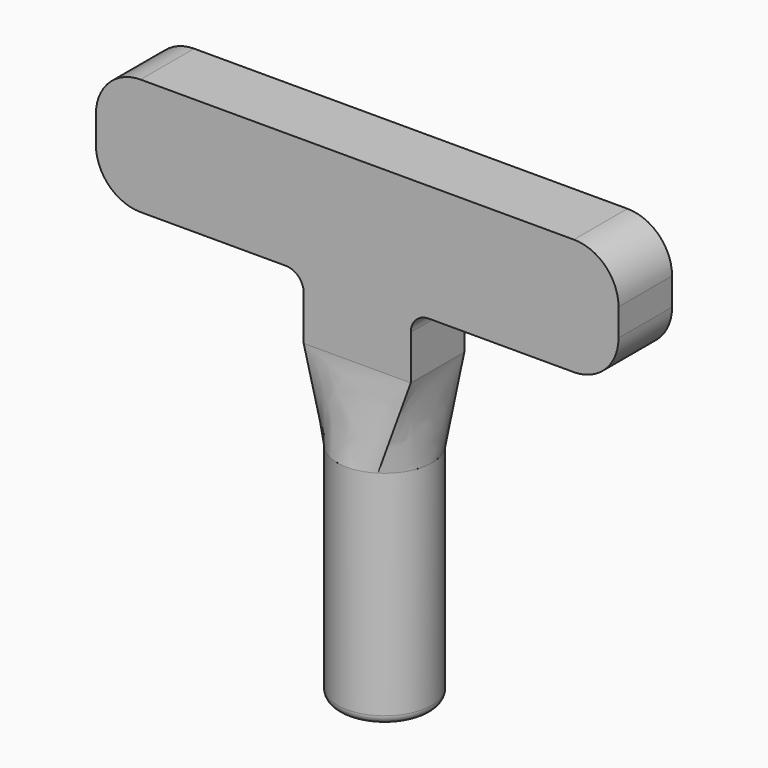
from build123d import *

# Parameters (mm, degrees)
F2_R      = 0.5
F4_DEPTH  = 7.5
F4_FACE_W = 24
F4_FACE_H = 15
F6_R      = 2


# Not quite as in the source:
# - the arcs of a loft's sections are written as splines that run evenly, so that the points pair up as in the source's solid


with BuildPart() as f1:
    # F0 (on Front) → F1 (revolve)
    with BuildSketch(Plane.XZ):
        Polygon((-7.6, -6.539241709), (-7.6, 9.460758291), (0, 9.460758291), (0, 43.2881079614), (-10.6, 43.2881079614), (-10.6, -6.539241709), align=None)
    revolve(axis=Axis((0, 0, 26.3744331262), (0, 0, -1)))

    # F2
    f2_edges = [f1.edges().sort_by_distance(p)[0] for p in [
        (7.6, 0, -6.539242),
    ]]
    fillet(f2_edges, radius=F2_R)

    # F6
    f6_edges = [f1.edges().sort_by_distance(p)[0] for p in [
        (10.6, 0, -6.539242),
        (8.1, 0, -6.539242),
    ]]
    fillet(f6_edges, radius=F6_R)


with BuildPart() as f4:
    # F3 (on Front) → F4 (new body, symmetric)
    with BuildSketch(Plane.XZ):
        with BuildLine():
            Line((-12.1438586622, 62.5112550155), (-0.1438586622, 62.5112550155))
            Line((-0.1438586622, 62.5112550155), (-0.1438586622, 102.6653030368))
            Line((-0.1438586622, 102.6653030368), (-48.6952245638, 102.6653030368))
            ThreePointArc((-48.6952245638, 102.6653030368), (-55.7662923757, 99.7363708486), (-58.6952245638, 92.6653030368))
            Line((-58.6952245638, 92.6653030368), (-58.6952245638, 86.5112550155))
            ThreePointArc((-58.6952245638, 86.5112550155), (-55.7662923757, 79.4401872036), (-48.6952245638, 76.5112550155))
            Line((-48.6952245638, 76.5112550155), (-16.1438586622, 76.5112550155))
            ThreePointArc((-16.1438586622, 76.5112550155), (-13.3154315374, 75.3396821402), (-12.1438586622, 72.5112550155))
            Line((-12.1438586622, 72.5112550155), (-12.1438586622, 62.5112550155))
        make_face()
        with BuildLine():
            Line((-0.1438586622, 102.6653030368), (-0.1438586622, 62.5112550155))
            Line((-0.1438586622, 62.5112550155), (11.8561413378, 62.5112550155))
            Line((11.8561413378, 62.5112550155), (11.8561413378, 72.5112550155))
            ThreePointArc((11.8561413378, 72.5112550155), (13.0277142131, 75.3396821402), (15.8561413378, 76.5112550155))
            Line((15.8561413378, 76.5112550155), (48.4075072394, 76.5112550155))
            ThreePointArc((48.4075072394, 76.5112550155), (55.4785750513, 79.4401872036), (58.4075072394, 86.5112550155))
            Line((58.4075072394, 86.5112550155), (58.4075072394, 92.6653030368))
            ThreePointArc((58.4075072394, 92.6653030368), (55.4785750513, 99.7363708486), (48.4075072394, 102.6653030368))
            Line((48.4075072394, 102.6653030368), (-0.1438586622, 102.6653030368))
        make_face()
    extrude(amount=F4_DEPTH, both=True)

    # F4_face (on face) → F5 section 0
    with BuildSketch(Plane(origin=(-0.1438586622, 0, 62.5112550155), x_dir=(1, 0, 0), z_dir=(0, 0, -1))):
        Rectangle(F4_FACE_W, F4_FACE_H)
    # F1_face (on face) → F5 section 1
    with BuildSketch(Plane.XY.offset(43.2881079614)):
        with BuildLine():
            add(Edge.make_bspline(
                [(8.9581169834, 5.6667574602), (8.2163401664, 6.8393722312), (7.2416993998, 7.8640350998), (4.9735940712, 9.463013276), (3.6810219119, 10.0366994541), (0.9736633644, 10.645996332), (-0.4400577936, 10.6813672994), (-3.1744987633, 10.2082229526), (-4.4941426892, 9.6998938003), (-5.6667574602, 8.9581169834)],
                knots=[0, 0, 0, 0, 0.25, 0.25, 0.5, 0.5, 0.75, 0.75, 1, 1, 1, 1], degree=3))
            add(Edge.make_bspline(
                [(-5.6667574602, 8.9581169834), (-6.8393722312, 8.2163401664), (-7.8640350998, 7.2416993998), (-9.463013276, 4.9735940712), (-10.0366994541, 3.6810219119), (-10.645996332, 0.9736633644), (-10.6813672994, -0.4400577936), (-10.2082229526, -3.1744987633), (-9.6998938003, -4.4941426892), (-8.9581169834, -5.6667574602)],
                knots=[0, 0, 0, 0, 0.25, 0.25, 0.5, 0.5, 0.75, 0.75, 1, 1, 1, 1], degree=3))
            add(Edge.make_bspline(
                [(-8.9581169834, -5.6667574602), (-8.2163401664, -6.8393722312), (-7.2416993998, -7.8640350998), (-4.9735940712, -9.463013276), (-3.6810219119, -10.0366994541), (-0.9736633644, -10.645996332), (0.4400577936, -10.6813672994), (3.1744987633, -10.2082229526), (4.4941426892, -9.6998938003), (5.6667574602, -8.9581169834)],
                knots=[0, 0, 0, 0, 0.25, 0.25, 0.5, 0.5, 0.75, 0.75, 1, 1, 1, 1], degree=3))
            add(Edge.make_bspline(
                [(5.6667574602, -8.9581169834), (6.8393722312, -8.2163401664), (7.8640350998, -7.2416993998), (9.463013276, -4.9735940712), (10.0366994541, -3.6810219119), (10.645996332, -0.9736633644), (10.6813672994, 0.4400577936), (10.2082229526, 3.1744987633), (9.6998938003, 4.4941426892), (8.9581169834, 5.6667574602)],
                knots=[0, 0, 0, 0, 0.25, 0.25, 0.5, 0.5, 0.75, 0.75, 1, 1, 1, 1], degree=3))
        make_face()
    loft(ruled=True)


solid = Compound([f1.part, f4.part])
